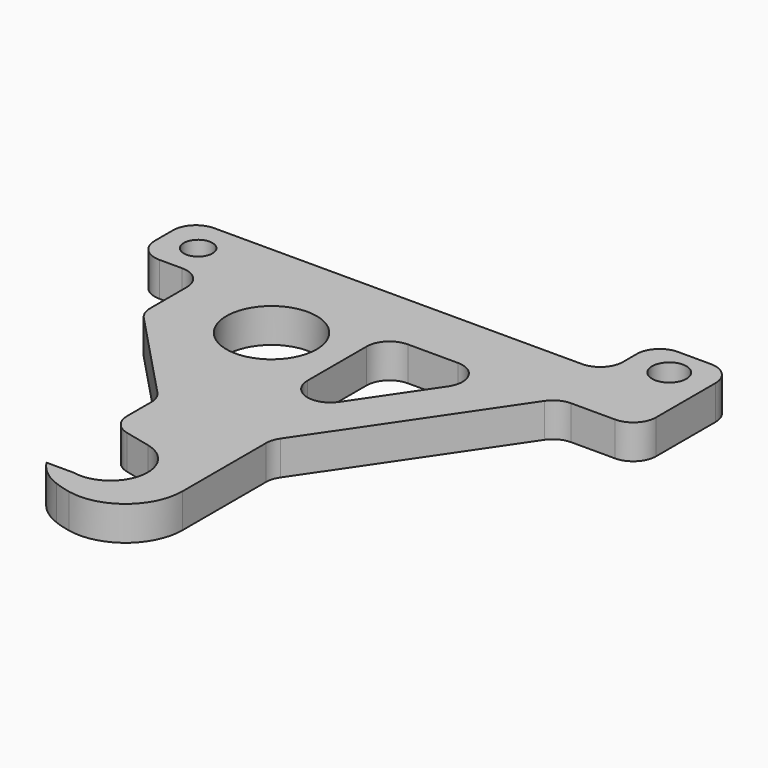
from build123d import *

# Parameters (mm, degrees)
F0_R        = 3.95
F0_R_2      = 1.25
F0_R_3      = 1.5
F1_DEPTH    = 3
F2_R        = 10
F3_R        = 2
F4_T1_DEPTH = 16.2671931878
F4_T3_DEPTH = 33.1863063341


# Not quite as in the source:
# - a fillet or chamfer that OpenCascade refuses, or shapes differently, is made with other operations: its cross-section is extruded or revolved along the edge and cut away or added
# - a feature names something its author has since deleted; it is built from what else it names


with BuildPart() as f1:
    # F0 (on Top) → F1 (new body)
    with BuildSketch(Plane.XY):
        with BuildLine():
            Line((4.0200765709, -14.8563961814), (9.9142113018, -14.8563961814))
            Line((9.9142113018, -14.8563961814), (9.9142113018, -11.4412054596))
            Line((9.9142113018, -11.4412054596), (9.9142113018, 0))
            Line((9.9142113018, 0), (21.4632351379, 17.0130324811))
            Line((21.4632351379, 17.0130324811), (28.3592351379, 17.0130324811))
            Line((28.3592351379, 17.0130324811), (28.3592351379, 22.0130324811))
            Line((28.3592351379, 22.0130324811), (28.3592351379, 27.5130324811))
            Line((28.3592351379, 27.5130324811), (21.4632351379, 27.5130324811))
            Line((21.4632351379, 27.5130324811), (21.4632351379, 22.0130324811))
            Line((21.4632351379, 22.0130324811), (-8.7310690433, 22.0130324811))
            Line((-8.7310690433, 22.0130324811), (-14.7310690433, 22.0130324811))
            Line((-14.7310690433, 22.0130324811), (-14.7310690433, 16.0130324811))
            Line((-14.7310690433, 16.0130324811), (-8.7310690433, 16.0130324811))
            Line((-8.7310690433, 16.0130324811), (-8.7310690433, 9.2081045732))
            Line((-8.7310690433, 9.2081045732), (0, 0))
            Line((0, 0), (0, -4.9987894588))
            Line((0, -4.9987894588), (3.805913418, -5.8956493604))
            ThreePointArc((3.805913418, -5.8956493604), (6.3099596188, -9.1166975853), (3.693151613, -12.2468277588))
            ThreePointArc((3.693151613, -12.2468277588), (3.0604717322, -12.3090046508), (2.4277918514, -12.2468277588))
            Line((2.4277918514, -12.2468277588), (0, -12.2468277588))
            Line((0, -12.2468277588), (0, -13.2468277588))
            Line((0, -13.2468277588), (4.0200765709, -14.8563961814))
        make_face()
        with Locations((0, 12.3804118484)):
            Circle(F0_R, mode=Mode.SUBTRACT)
        with Locations((-11.7310690433, 19.0130324811)):
            Circle(F0_R_2, mode=Mode.SUBTRACT)
        Polygon((6.3511028036, 16.8475485612), (16.5163309854, 16.8475485612), (6.3511028036, 1.8730052848), align=None, mode=Mode.SUBTRACT)
        with Locations((24.9112351379, 24.7630324811)):
            Circle(F0_R_3, mode=Mode.SUBTRACT)
    extrude(amount=F1_DEPTH)

    # F2
    f2_edges = [f1.edges().sort_by_distance(p)[0] for p in [
        (4.020077, -14.856396, 1.5),
    ]]
    fillet(f2_edges, radius=F2_R)

    # F3
    f3_edges = [f1.edges().sort_by_distance(p)[0] for p in [
        (21.463235, 22.013032, 1.5),
        (-8.731069, 9.208105, 1.5),
        (21.463235, 17.013032, 1.5),
        (0, 0, 1.5),
        (0, -4.998789, 1.5),
        (9.914211, 0, 1.5),
        (6.351103, 16.847549, 1.5),
        (16.516331, 16.847549, 1.5),
        (6.351103, 1.873005, 1.5),
        (-14.731069, 16.013032, 1.5),
        (-14.731069, 22.013032, 1.5),
        (28.359235, 27.513032, 1.5),
        (21.463235, 27.513032, 1.5),
        (28.359235, 17.013032, 1.5),
        (-8.731069, 16.013032, 1.5),
    ]]
    fillet(f3_edges, radius=F3_R)

    # F4: fillet of radius 5 on 2 edges, made by hand

    # F4_s2 → F4_t1 (cut)
    with BuildSketch(Plane.XY.offset(-6.6335965939)):
        with BuildLine():
            ThreePointArc((2.4644968667, -14.2301851696), (1.0712579431, -13.4385513762), (0, -12.2468277588))
            Line((0, -12.2468277588), (-0.4206053642, -12.5171814672))
            ThreePointArc((-0.4206053642, -12.5171814672), (-0.5, -12.7468277588), (-0.5, -13.2468277588))
            Line((-0.5, -13.2468277588), (-0.1858483979, -13.7110048511))
            ThreePointArc((-0.1858483979, -13.7110048511), (2.0447940609, -14.6041151192), (2.2903411892, -14.698874619))
            Line((2.2903411892, -14.698874619), (2.4644968667, -14.2301851696))
        make_face()
    extrude(amount=F4_T1_DEPTH, mode=Mode.SUBTRACT)

    # F4_s4 → F4_t3 (cut)
    with BuildSketch(Plane.XY.offset(-15.0931531671)):
        with BuildLine():
            ThreePointArc((9.9142113018, -9.7484393403), (8.063259128, -13.6321872452), (3.8808121864, -14.6404824992))
            Line((3.8808121864, -14.6404824992), (3.7774722749, -15.1296868151))
            ThreePointArc((3.7774722749, -15.1296868151), (5.9476104172, -15.3563961814), (9.9142113018, -15.3563961814))
            Line((9.9142113018, -15.3563961814), (10.4142113018, -14.8563961814))
            Line((10.4142113018, -14.8563961814), (10.4142113018, -9.7484393403))
            Line((10.4142113018, -9.7484393403), (9.9142113018, -9.7484393403))
        make_face()
    extrude(amount=F4_T3_DEPTH, mode=Mode.SUBTRACT)


solid = f1.part
